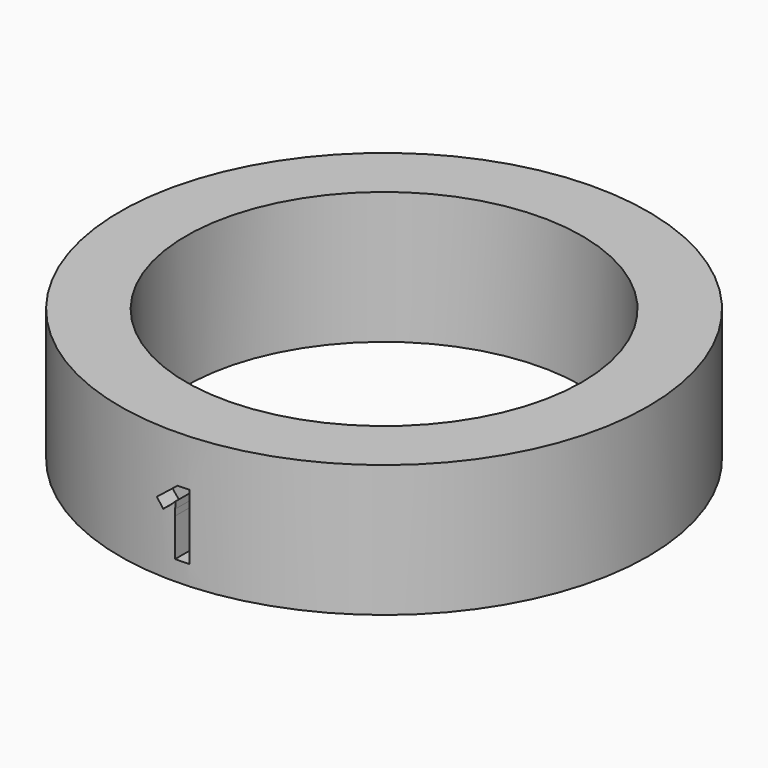
from build123d import *

# Parameters (mm, degrees)
F0_R         = 20
F0_R_2       = 15
F1_DEPTH     = 10
F3_TEXT_SIZE = 6.9444444444
F4_DEPTH     = 1.5


# Not quite as in the source:
# - Text() gives the source's letters only with a copy of the font that has no kerning and outlines rounded to 1/6400 em; it was checked with that copy


with BuildPart() as f1:
    # F0 (on Top) → F1 (new body)
    with BuildSketch(Plane.XY):
        Circle(F0_R)
        Circle(F0_R_2, mode=Mode.SUBTRACT)
    extrude(amount=F1_DEPTH)

    # F3 (on offset) → F4 (cut)
    with BuildSketch(Plane.XZ.offset(20)):
        with Locations((-1.6596137153, 1.5)):
            Text('1', F3_TEXT_SIZE, font='Open Sans', font_style=FontStyle.BOLD, text_align=(TextAlign.LEFT, TextAlign.BOTTOM))
    extrude(amount=-F4_DEPTH, mode=Mode.SUBTRACT)


solid = f1.part
